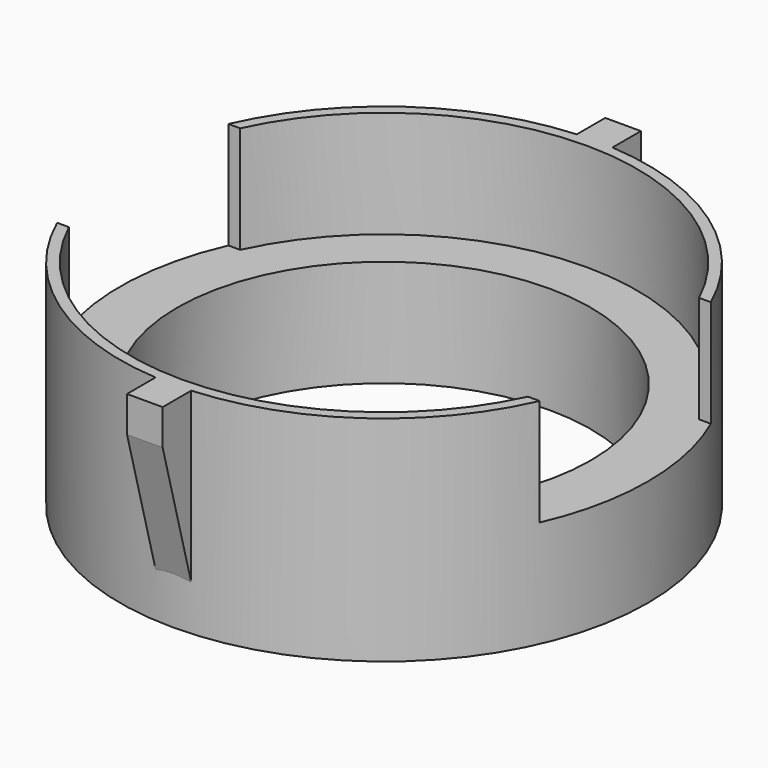
from build123d import *

# Parameters (mm, degrees)
F0_R         = 37
F0_R_2       = 35.5
F1_DEPTH     = 30
F2_W         = 100
F2_H         = 30
F3_DEPTH     = 15
F6_R         = 35.5
F6_R_2       = 29
F7_DEPTH     = 15
F8_W         = 5
F8_H         = 5
F9_DEPTH     = 25
F10_T4_DEPTH = 108.868862808
F10_S5_R     = 37
F10_T6_DEPTH = 57
F11_W        = 5
F11_H        = 5
F12_DEPTH    = 25
F13_T4_DEPTH = 108.868862808
F13_S5_R     = 37
F13_T6_DEPTH = 57


# Not quite as in the source:
# - a fillet or chamfer that OpenCascade refuses, or shapes differently, is made with other operations: its cross-section is extruded or revolved along the edge and cut away or added


with BuildPart() as f1:
    # F0 (on Top) → F1 (new body)
    with BuildSketch(Plane.XY):
        Circle(F0_R)
        Circle(F0_R_2, mode=Mode.SUBTRACT)
    extrude(amount=F1_DEPTH)


with BuildPart() as f3:
    # F2 (on Top) → F3 (new body)
    with BuildSketch(Plane.XY):
        Rectangle(F2_W, F2_H)
    extrude(amount=F3_DEPTH)


with BuildPart() as f3_1:
    # F4: moved
    add(f3.part.moved(Location((0, 0, 15))))


with BuildPart() as f1_1:
    add(f1.part)

    # F5: cut F3
    add(f3_1.part, mode=Mode.SUBTRACT)

    # F6 (on Top) → F7 (join)
    with BuildSketch(Plane.XY):
        Circle(F6_R)
        Circle(F6_R_2, mode=Mode.SUBTRACT)
    extrude(amount=F7_DEPTH)

    # F8 (on face) → F9 (join)
    with BuildSketch(Plane.XY.offset(30)):
        with Locations((0, -39.4154439226)):
            Rectangle(F8_W, F8_H)
    extrude(amount=-F9_DEPTH)

    # F10: chamfer of 20 x 5.3589838486 on 1 edges, made by hand


with BuildPart() as f10_tool2:
    # F10_s3 → F10_t4 (new body)
    with BuildSketch(Plane.YZ.offset(-54.434431404)):
        Polygon((-36.5564600739, 5), (-41.9154439226, 25), (-41.9154439226, 5), align=None)
    extrude(amount=F10_T4_DEPTH)

    # F10_s5 → F10_t6 (cut, symmetric)
    with BuildSketch(Plane.XY.offset(15)):
        Circle(F10_S5_R)
    extrude(amount=F10_T6_DEPTH, both=True, mode=Mode.SUBTRACT)


with BuildPart() as f1_2:
    add(f1_1.part)

    # F10_t1: cut F10_tool2
    add(f10_tool2.part, mode=Mode.SUBTRACT)

    # F11 (on face) → F12 (join)
    with BuildSketch(Plane.XY.offset(30)):
        with Locations((0, 39.3967875838)):
            Rectangle(F11_W, F11_H)
    extrude(amount=-F12_DEPTH)

    # F13: chamfer of 20 x 5.3589838486 on 1 edges, made by hand


with BuildPart() as f13_tool2:
    # F13_s3 → F13_t4 (new body)
    with BuildSketch(Plane.YZ.offset(54.434431404)):
        Polygon((36.5378037352, 5), (41.8967875838, 25), (41.8967875838, 5), align=None)
    extrude(amount=-F13_T4_DEPTH)

    # F13_s5 → F13_t6 (cut, symmetric)
    with BuildSketch(Plane.XY.offset(15)):
        Circle(F13_S5_R)
    extrude(amount=F13_T6_DEPTH, both=True, mode=Mode.SUBTRACT)


with BuildPart() as f1_3:
    add(f1_2.part)

    # F13_t1: cut F13_tool2
    add(f13_tool2.part, mode=Mode.SUBTRACT)


solid = f1_3.part
